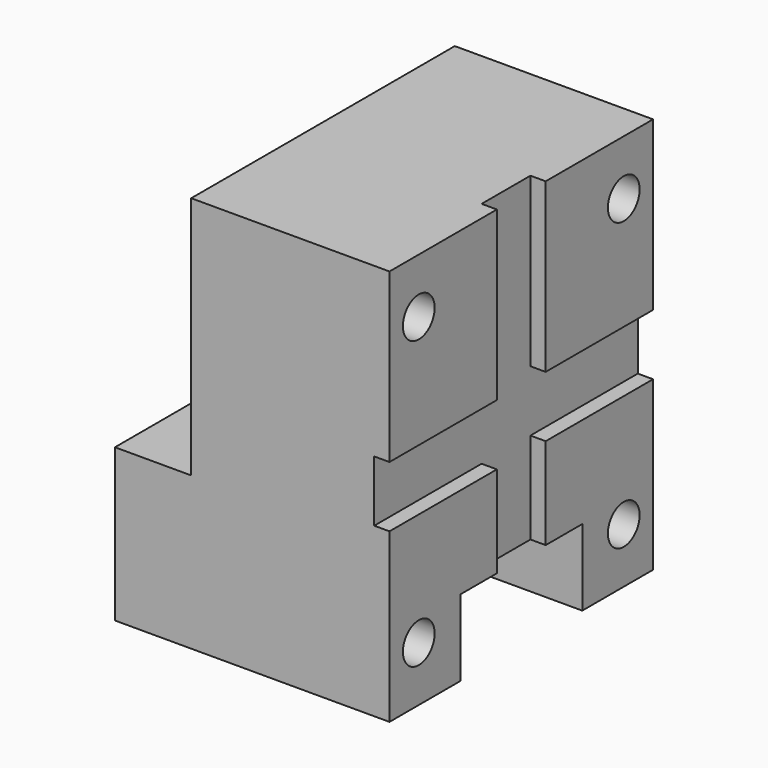
from build123d import *

# Parameters (mm, degrees)
F0_W      = 108
F0_H      = 130
F1_DEPTH  = 90
F2_R      = 6.5
F3_DEPTH  = 90.001
F4_W      = 108
F4_H      = 80
F5_DEPTH  = 25
F6_W      = 90
F6_H      = 50
F7_DEPTH  = 25
F8_R      = 10
F9_DEPTH  = 20
F10_R     = 10
F11_DEPTH = 20
F12_W     = 20
F12_H     = 55
F12_W_2   = 44
F12_H_2   = 20
F13_DEPTH = 5
F15_ANGLE = 180


with BuildPart() as f1:
    # F0 (on Right) → F1 (new body)
    with BuildSketch(Plane.YZ):
        Rectangle(F0_W, F0_H)
    extrude(amount=-F1_DEPTH)

    # F2 (on face) → F3 (cut, through all)
    with BuildSketch(Plane(origin=(-90, 0, 0), x_dir=(0, -1, 0), z_dir=(-1, 0, 0))):
        with Locations((-42, 47)):
            Circle(F2_R)
        with Locations((42, 47)):
            Circle(F2_R)
        with Locations((-42, -47)):
            Circle(F2_R)
        with Locations((42, -47)):
            Circle(F2_R)
    extrude(amount=-F3_DEPTH, mode=Mode.SUBTRACT)

    # F4 (on face) → F5 (cut)
    with BuildSketch(Plane(origin=(-90, 0, 0), x_dir=(0, -1, 0), z_dir=(-1, 0, 0))):
        with Locations((0, -25)):
            Rectangle(F4_W, F4_H)
    extrude(amount=-F5_DEPTH, mode=Mode.SUBTRACT)

    # F6 (on face) → F7 (cut)
    with BuildSketch(Plane.XY.offset(65)):
        with Locations((-45, 0)):
            Rectangle(F6_W, F6_H)
    extrude(amount=-F7_DEPTH, mode=Mode.SUBTRACT)

    # F8 (on face) → F9 (cut)
    with BuildSketch(Plane(origin=(-65, 0, 0), x_dir=(0, -1, 0), z_dir=(-1, 0, 0))):
        with Locations((42, -47)):
            Circle(F8_R)
        with Locations((-42, -47)):
            Circle(F8_R)
    extrude(amount=-F9_DEPTH, mode=Mode.SUBTRACT)

    # F10 (on face) → F11 (cut)
    with BuildSketch(Plane(origin=(-90, 0, 0), x_dir=(0, -1, 0), z_dir=(-1, 0, 0))):
        with Locations((42, 47)):
            Circle(F10_R)
        with Locations((-42, 47)):
            Circle(F10_R)
    extrude(amount=-F11_DEPTH, mode=Mode.SUBTRACT)

    # F12 (on face) → F13 (cut)
    with BuildSketch(Plane.YZ):
        with Locations((0, -37.5)):
            Rectangle(F12_W, F12_H)
        with Locations((-32, 0)):
            Rectangle(F12_W_2, F12_H_2)
        Rectangle(F12_W, F12_H_2)
        with Locations((32, 0)):
            Rectangle(F12_W_2, F12_H_2)
        with Locations((0, 37.5)):
            Rectangle(F12_W, F12_H)
    extrude(amount=-F13_DEPTH, mode=Mode.SUBTRACT)


with BuildPart() as f1_1:
    # F15: moved
    add(f1.part.rotate(Axis((42.7994653583, 0, 0), (1, 0, 0)), F15_ANGLE))


solid = f1_1.part
